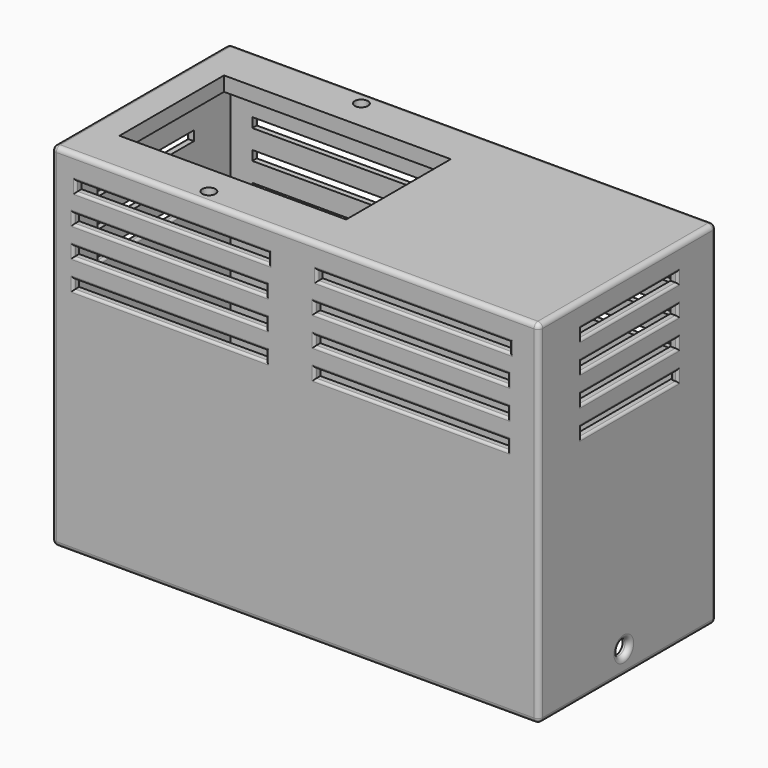
from build123d import *

# Parameters (mm, degrees)
F0_W          = 101
F0_H          = 46
F0_W_2        = 98
F0_H_2        = 43
F1_DEPTH      = 73
F0_R          = 1.375
F0_W_3        = 47
F0_H_3        = 27.1
F0_W_4        = 13
F0_H_4        = 20
F2_DEPTH      = 3
F4_R          = 1.55
F5_DEPTH      = 3
F6_R          = 1
F8_W          = 40
F8_H          = 2
F9_DEPTH      = 3
F7_W          = 40
F7_H          = 2
F10_DEPTH     = 3
F11_W         = 25
F11_H         = 2
F12_DEPTH     = 3
F13_W         = 25
F13_H         = 2
F14_DEPTH     = 3
F15_R         = 0.5
F16_TEXT_SIZE = 9.3799860527
F17_DEPTH     = 0.75
F18_DEPTH     = 3


# Not quite as in the source:
# - Text() gives the source's letters only with a copy of the font that has no kerning and outlines rounded to 1/6400 em; it was checked with that copy


with BuildPart() as f1:
    # F0 (on Top) → F1 (new body)
    with BuildSketch(Plane.XY):
        Rectangle(F0_W, F0_H)
        Rectangle(F0_W_2, F0_H_2, mode=Mode.SUBTRACT)
    extrude(amount=-F1_DEPTH)

    # F0 (on Top) → F2 (join)
    with BuildSketch(Plane.XY):
        Rectangle(F0_W_2, F0_H_2)
        with Locations((-20.5, -19.75)):
            Circle(F0_R, mode=Mode.SUBTRACT)
        with Locations((-20.5, 0)):
            Rectangle(F0_W_3, F0_H_3, mode=Mode.SUBTRACT)
        with Locations((-20.5, 19.75)):
            Circle(F0_R, mode=Mode.SUBTRACT)
        with Locations((32.5, 0)):
            Rectangle(F0_W_4, F0_H_4, mode=Mode.SUBTRACT)
    extrude(amount=-F2_DEPTH)

    # F4 (on face) → F5 (cut)
    with BuildSketch(Plane.YZ.offset(50.5)):
        with Locations((-1, -68)):
            Circle(F4_R)
    extrude(amount=-F5_DEPTH, mode=Mode.SUBTRACT)

    # F6
    f6_edges = [f1.edges().sort_by_distance(p)[0] for p in [
        (0, -23, -73),
        (50.5, 0, -73),
        (0, 23, -73),
        (-50.5, 0, -73),
        (-50.5, -23, -36.5),
        (-50.5, 23, -36.5),
        (50.5, -23, -36.5),
        (50.5, 23, -36.5),
        (0, -23, 0),
        (50.5, 0, 0),
        (0, 23, 0),
        (-50.5, 0, 0),
        (50.5, -2.55, -68),
    ]]
    fillet(f6_edges, radius=F6_R)

    # F8 (on face) → F9 (cut)
    with BuildSketch(Plane(origin=(0, 23, 0), x_dir=(-1, 0, 0), z_dir=(0, 1, 0))):
        with Locations((24.5, -6)):
            Rectangle(F8_W, F8_H)
        with Locations((-25.5, -6)):
            Rectangle(F8_W, F8_H)
        with Locations((24.5, -12)):
            Rectangle(F8_W, F8_H)
        with Locations((-25.5, -12)):
            Rectangle(F8_W, F8_H)
        with Locations((24.5, -18)):
            Rectangle(F8_W, F8_H)
        with Locations((-25.5, -18)):
            Rectangle(F8_W, F8_H)
        with Locations((24.5, -24)):
            Rectangle(F8_W, F8_H)
        with Locations((-25.5, -24)):
            Rectangle(F8_W, F8_H)
    extrude(amount=-F9_DEPTH, mode=Mode.SUBTRACT)

    # F7 (on face) → F10 (cut)
    with BuildSketch(Plane.XZ.offset(23)):
        with Locations((24.5, -6)):
            Rectangle(F7_W, F7_H)
        with Locations((-25.5, -6)):
            Rectangle(F7_W, F7_H)
        with Locations((24, -12)):
            Rectangle(F7_W, F7_H)
        with Locations((-26, -12)):
            Rectangle(F7_W, F7_H)
        with Locations((24, -18)):
            Rectangle(F7_W, F7_H)
        with Locations((-26, -18)):
            Rectangle(F7_W, F7_H)
        with Locations((24, -24)):
            Rectangle(F7_W, F7_H)
        with Locations((-26, -24)):
            Rectangle(F7_W, F7_H)
    extrude(amount=-F10_DEPTH, mode=Mode.SUBTRACT)

    # F11 (on face) → F12 (cut)
    with BuildSketch(Plane.YZ.offset(50.5)):
        with Locations((0.5, -6)):
            Rectangle(F11_W, F11_H)
        with Locations((0.5, -12)):
            Rectangle(F11_W, F11_H)
        with Locations((0.5, -18)):
            Rectangle(F11_W, F11_H)
        with Locations((0.5, -24)):
            Rectangle(F11_W, F11_H)
    extrude(amount=-F12_DEPTH, mode=Mode.SUBTRACT)

    # F13 (on face) → F14 (cut)
    with BuildSketch(Plane(origin=(-50.5, 0, 0), x_dir=(0, -1, 0), z_dir=(-1, 0, 0))):
        with Locations((0.5, -6)):
            Rectangle(F13_W, F13_H)
        with Locations((0.5, -12)):
            Rectangle(F13_W, F13_H)
        with Locations((0.5, -18)):
            Rectangle(F13_W, F13_H)
        with Locations((0.5, -24)):
            Rectangle(F13_W, F13_H)
    extrude(amount=-F14_DEPTH, mode=Mode.SUBTRACT)

    # F15
    f15_edges = [f1.edges().sort_by_distance(p)[0] for p in [
        (44, -23, -24),
        (24, -23, -25),
        (24, -23, -23),
        (4, -23, -24),
        (24, -23, -19),
        (44, -23, -18),
        (24, -23, -17),
        (4, -23, -18),
        (4, -23, -12),
        (24, -23, -13),
        (44, -23, -12),
        (24, -23, -11),
        (24.5, -23, -7),
        (44.5, -23, -6),
        (24.5, -23, -5),
        (4.5, -23, -6),
        (-6, -23, -24),
        (-26, -23, -25),
        (-46, -23, -24),
        (-26, -23, -23),
        (-26, -23, -19),
        (-6, -23, -18),
        (-26, -23, -17),
        (-46, -23, -18),
        (-46, -23, -12),
        (-26, -23, -13),
        (-6, -23, -12),
        (-26, -23, -11),
        (-25.5, -23, -7),
        (-5.5, -23, -6),
        (-25.5, -23, -5),
        (-45.5, -23, -6),
        (50.5, 0.5, -25),
        (49, 13, -24),
        (50.5, 0.5, -23),
        (50.5, -12, -24),
        (50.5, -12, -18),
        (50.5, 0.5, -19),
        (50.5, 13, -18),
        (50.5, 0.5, -17),
        (50.5, 13, -12),
        (50.5, 0.5, -13),
        (50.5, 0.5, -11),
        (50.5, -12, -12),
        (50.5, -12, -6),
        (50.5, 0.5, -7),
        (50.5, 13, -6),
        (50.5, 0.5, -5),
        (50.5, 13, -24),
        (25.5, 23, -25),
        (5.5, 23, -24),
        (45.5, 23, -24),
        (25.5, 23, -23),
        (25.5, 23, -19),
        (45.5, 23, -18),
        (25.5, 23, -17),
        (5.5, 23, -18),
        (5.5, 23, -12),
        (25.5, 23, -13),
        (25.5, 23, -11),
        (45.5, 23, -12),
        (45.5, 23, -6),
        (25.5, 23, -7),
        (25.5, 23, -5),
        (5.5, 23, -6),
        (-4.5, 23, -24),
        (-24.5, 23, -25),
        (-44.5, 23, -24),
        (-24.5, 23, -23),
        (-24.5, 23, -19),
        (-44.5, 23, -18),
        (-24.5, 23, -17),
        (-4.5, 23, -18),
        (-4.5, 23, -12),
        (-24.5, 23, -13),
        (-24.5, 23, -11),
        (-44.5, 23, -12),
        (-44.5, 23, -6),
        (-24.5, 23, -7),
        (-24.5, 23, -5),
        (-4.5, 23, -6),
        (-50.5, -0.5, -5),
        (-50.5, -0.5, -7),
        (-50.5, 12, -6),
        (-50.5, -13, -6),
        (-50.5, -13, -12),
        (-50.5, -0.5, -13),
        (-50.5, -0.5, -11),
        (-50.5, 12, -12),
        (-50.5, -0.5, -17),
        (-50.5, 12, -18),
        (-50.5, -0.5, -19),
        (-50.5, -13, -18),
        (-50.5, -0.5, -23),
        (-49, -0.5, -25),
        (-50.5, 12, -24),
        (-50.5, -0.5, -25),
        (-50.5, -13, -24),
    ]]
    fillet(f15_edges, radius=F15_R)

    # F16 (on face) → F17 (cut)
    with BuildSketch(Plane(origin=(-50.5, 0, 0), x_dir=(0, -1, 0), z_dir=(-1, 0, 0))):
        with Locations((-6.9646397606, -39.2712727189)):
            Text('idk', F16_TEXT_SIZE, font='Open Sans', font_style=FontStyle.BOLD, text_align=(TextAlign.LEFT, TextAlign.BOTTOM))
    extrude(amount=-F17_DEPTH, mode=Mode.SUBTRACT)

    # F0 (on Top) → F18 (join)
    with BuildSketch(Plane.XY):
        with Locations((32.5, 0)):
            Rectangle(F0_W_4, F0_H_4)
    extrude(amount=-F18_DEPTH)


solid = f1.part
